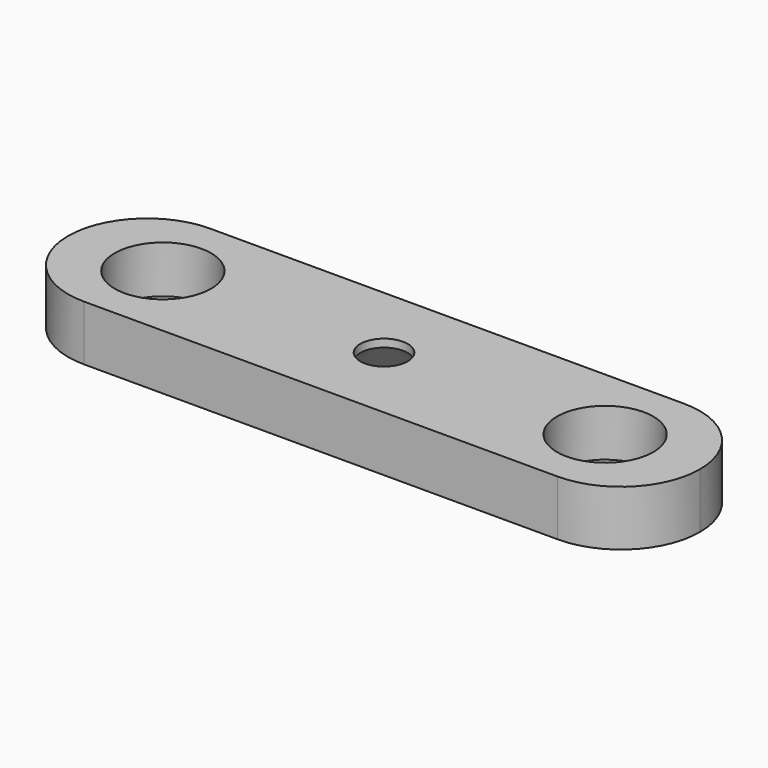
from build123d import *

# Parameters (mm, degrees)
F0_W     = 40
F0_H     = 10
F0_R     = 3.05
F0_R_2   = 1.5
F1_DEPTH = 0.5
F2_DEPTH = 3.5
F3_R     = 4.99999
F4_SIZE  = 3


# Not quite as in the source:
# - a fillet or chamfer is up to 0.001 mm smaller than in the source, because OpenCascade refuses the exact size


with BuildPart() as f1:
    # F0 (on Top) → F1 (new body)
    with BuildSketch(Plane.XY):
        Rectangle(F0_W, F0_H)
        with Locations((-14, 0)):
            Circle(F0_R, mode=Mode.SUBTRACT)
        Circle(F0_R_2, mode=Mode.SUBTRACT)
        with Locations((14, 0)):
            Circle(F0_R, mode=Mode.SUBTRACT)
        with Locations((-14, 0)):
            Circle(F0_R)
        with Locations((14, 0)):
            Circle(F0_R)
    extrude(amount=F1_DEPTH)

    # F0 (on Top) → F2 (join)
    with BuildSketch(Plane.XY):
        Rectangle(F0_W, F0_H)
        with Locations((-14, 0)):
            Circle(F0_R, mode=Mode.SUBTRACT)
        Circle(F0_R_2, mode=Mode.SUBTRACT)
        with Locations((14, 0)):
            Circle(F0_R, mode=Mode.SUBTRACT)
    extrude(amount=F2_DEPTH)

    # F3 (radius 5 in the source; OpenCascade refuses exactly that, so slightly less here)
    f3_edges = [f1.edges().sort_by_distance(p)[0] for p in [
        (20, 5, 1.75),
        (20, -5, 1.75),
        (-20, -5, 1.75),
        (-20, 5, 1.75),
    ]]
    fillet(f3_edges, radius=F3_R)

    # F4
    f4_edges = [f1.edges().sort_by_distance(p)[0] for p in [
        (-1.5, 0, 0),
    ]]
    chamfer(f4_edges, length=F4_SIZE)


solid = f1.part
